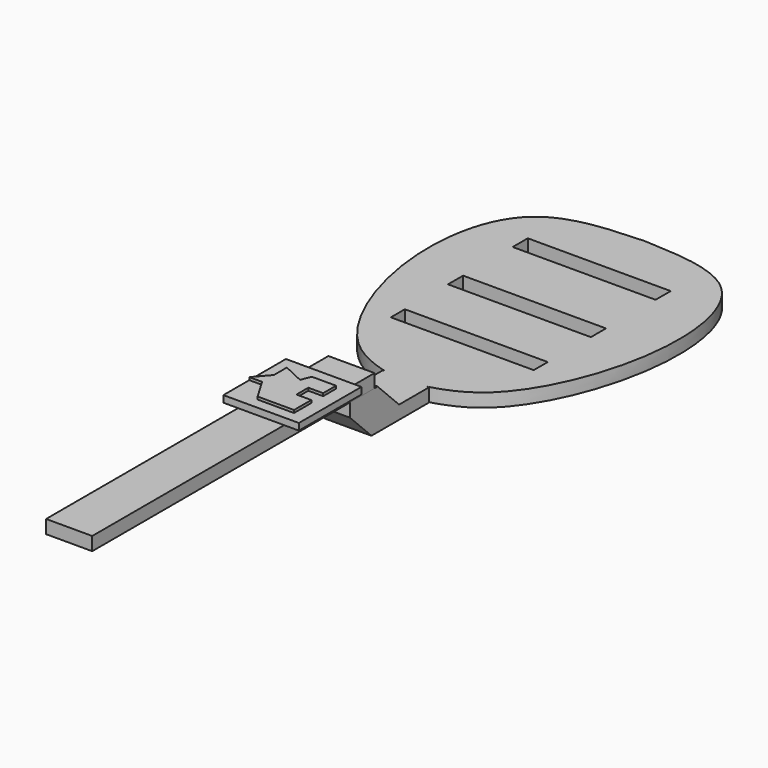
from build123d import *

# Parameters (mm, degrees)
F0_W     = 27.0528234541
F0_H     = 3.3177994192
F0_H_2   = 3.5730116069
F0_H_3   = 3.5730153322
F1_DEPTH = 2.54
F0_W_2   = 8.7334977924
F0_H_4   = 11.6122970358
F2_DEPTH = 7.62
F4_DEPTH = 2.54
F5_SIZE  = 5.07999
F6_W     = 14.2920585349
F6_H     = 14.8024894297
F7_DEPTH = 1.27
F9_DEPTH = 0.508


# Not quite as in the source:
# - a fillet or chamfer is up to 0.001 mm smaller than in the source, because OpenCascade refuses the exact size


with BuildPart() as f1:
    # F0 (on Top) → F1 (new body)
    with BuildSketch(Plane.XY):
        with BuildLine():
            add(Edge.make_bspline(
                [(0, 63.577234745), (6.943171273, 63.2683845738), (21.5991155841, 62.6164503593), (25.9966448984, 35.8068070443), (15.8071406297, 11.5475044882), (6.9938303995, 7.9173166599), (4.0047332195, 7.0992700308)],
                knots=[0, 0, 0, 0, 0.2400386989, 0.5066840016, 0.7952644813, 0.9371547504, 0.9371547504, 0.9371547504, 0.9371547504], degree=3))
            add(Edge.make_bspline(
                [(0, 63.577234745), (-6.943171273, 63.2683845738), (-21.5991155841, 62.6164503593), (-25.9966448984, 35.8068070443), (-15.8071406297, 11.5475044882), (-6.9938303995, 7.9173166599), (-4.0047332195, 7.0992700308)],
                knots=[0, 0, 0, 0, 0.2400386989, 0.5066840016, 0.7952644813, 0.9371547504, 0.9371547504, 0.9371547504, 0.9371547504], degree=3))
            Line((-4.0047332195, 7.0992700308), (4.0047332195, 7.0992700308))
        make_face()
        with Locations((-0.5104308948, 22.714164108)):
            Rectangle(F0_W, F0_H, mode=Mode.SUBTRACT)
        with Locations((-0.5104308948, 36.368181929)):
            Rectangle(F0_W, F0_H_2, mode=Mode.SUBTRACT)
        with Locations((-0.5104308948, 51.6811013222)):
            Rectangle(F0_W, F0_H_3, mode=Mode.SUBTRACT)
        with BuildLine():
            Line((4.0047332195, 7.0992700308), (-4.0047332195, 7.0992700308))
            add(Edge.make_bspline(
                [(-4.0047332195, 7.0992700308), (-2.6808189042, 6.736945363), (-1.3404094521, 6.4488768122), (0, 6.1608082615)],
                knots=[0.9371547504, 0.9371547504, 0.9371547504, 0.9371547504, 1, 1, 1, 1], degree=3))
            add(Edge.make_bspline(
                [(4.0047332195, 7.0992700308), (2.6808189042, 6.736945363), (1.3404094521, 6.4488768122), (0, 6.1608082615)],
                knots=[0.9371547504, 0.9371547504, 0.9371547504, 0.9371547504, 1, 1, 1, 1], degree=3))
        make_face()
        with BuildLine():
            add(Edge.make_bspline(
                [(-4.0047332195, 7.0992700308), (-2.6808189042, 6.736945363), (-1.3404094521, 6.4488768122), (0, 6.1608082615)],
                knots=[0.9371547504, 0.9371547504, 0.9371547504, 0.9371547504, 1, 1, 1, 1], degree=3))
            Line((-4.0047332195, 7.0992700308), (-4.3667488962, 7.0992700308))
            Line((-4.3667488962, 7.0992700308), (-4.3667488962, 0))
            Line((-4.3667488962, 0), (4.3667488962, 0))
            Line((4.3667488962, 0), (4.3667488962, 7.0992700308))
            Line((4.3667488962, 7.0992700308), (4.0047332195, 7.0992700308))
            add(Edge.make_bspline(
                [(4.0047332195, 7.0992700308), (2.6808189042, 6.736945363), (1.3404094521, 6.4488768122), (0, 6.1608082615)],
                knots=[0.9371547504, 0.9371547504, 0.9371547504, 0.9371547504, 1, 1, 1, 1], degree=3))
        make_face()
    extrude(amount=F1_DEPTH)

    # F0 (on Top) → F2 (join)
    with BuildSketch(Plane.XY):
        with Locations((0, -5.8061485179)):
            Rectangle(F0_W_2, F0_H_4)
    extrude(amount=F2_DEPTH)

    # F5 (size 5.08 in the source; OpenCascade refuses exactly that, so slightly less here)
    f5_edges = [f1.edges().sort_by_distance(p)[0] for p in [
        (0, -11.612297, 0),
        (0, 0, 7.62),
    ]]
    chamfer(f5_edges, length=F5_SIZE)


with BuildPart() as f4:
    # F3 (on face) → F4 (new body)
    with BuildSketch(Plane.XY.offset(7.62)):
        Polygon((4.3667488962, -5.8061485179), (-4.3667488962, -5.8061485179), (-4.3667488962, -72.6087614894), (4.3667488962, -72.6087614894), (4.3667488962, -70.3118219972), align=None)
    extrude(amount=F4_DEPTH)

    # F6 (on face) → F7 (join)
    with BuildSketch(Plane.XY.offset(10.16)):
        with Locations((0, -19.7791866958)):
            Rectangle(F6_W, F6_H)
    extrude(amount=F7_DEPTH)

    # F8 (on face) → F9 (join)
    with BuildSketch(Plane.XY.offset(11.43)):
        Polygon((4.5938747935, -15.1853114367), (0, -15.1853114367), (-0.7342260891, -17.0616675849), (1.7865073169, -18.2478949428), (4.5938747935, -18.2478949428), align=None)
        Polygon((-2.2969373967, -21.0552643985), (-0.7342260891, -17.0616675849), (-4.7214833321, -15.1853114367), (-4.7214833321, -18.2478949428), (-7.1460292675, -21.0552643985), (-4.7214833321, -21.0552643985), align=None)
        Polygon((1.7865073169, -18.2478949428), (-0.7342260891, -17.0616675849), (-2.2969373967, -21.0552643985), (4.5938747935, -25.1387096941), (4.5938747935, -21.0552643985), (1.7865073169, -21.0552643985), align=None)
        Polygon((4.5938747935, -25.1387096941), (-2.2969373967, -21.0552643985), (-2.2969373967, -25.1387096941), align=None)
        Polygon((-2.2969373967, -25.1387096941), (-2.2969373967, -21.0552643985), (-4.7214833321, -21.0552643985), align=None)
    extrude(amount=F9_DEPTH)


solid = Compound([f1.part, f4.part])
